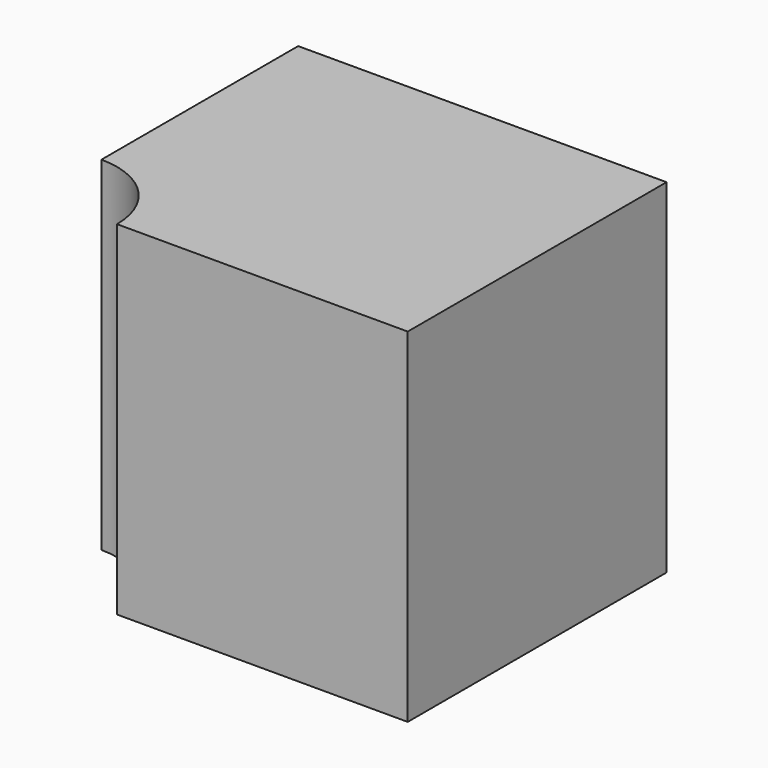
from build123d import *

# Parameters (mm, degrees)
F2_DEPTH = 70.7538053393


# Not quite as in the source:
# - a feature names something its author has since deleted; it is built from what else it names


with BuildPart() as f2:
    # F0 (on Top) → F2 (new body, through all)
    with BuildSketch(Plane.XY):
        with BuildLine():
            Line((37.9233248532, 33.3045050502), (-37.9233248532, 33.3045050502))
            Line((-37.9233248532, 33.3045050502), (-37.9233248532, -17.321989961))
            ThreePointArc((-37.9233248532, -17.321989961), (-26.6219800532, -22.0031602502), (-21.940809764, -33.3045050502))
            Line((-21.940809764, -33.3045050502), (37.9233248532, -33.3045050502))
            Line((37.9233248532, -33.3045050502), (37.9233248532, -14.8748438805))
            Line((37.9233248532, -14.8748438805), (37.9233248532, 16.9966574758))
            Line((37.9233248532, 16.9966574758), (37.9233248532, 33.3045050502))
        make_face()
    extrude(amount=F2_DEPTH)


solid = f2.part
